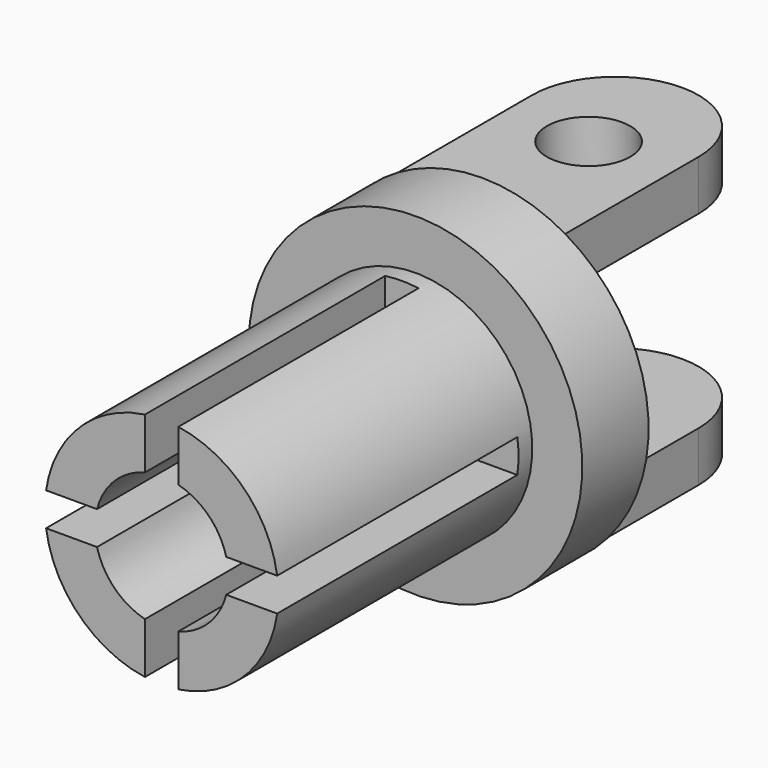
from build123d import *

# Parameters (mm, degrees)
F2_W     = 10
F2_H     = 3
F3_DEPTH = 15
F4_R     = 4.99999
F5_R     = 2.5
F6_DEPTH = 18.6612540378
F7_W     = 2
F7_H     = 4.8000003753
F7_W_2   = 4.8000003753
F7_H_2   = 2
F8_DEPTH = 18


# Not quite as in the source:
# - a fillet or chamfer is up to 0.001 mm smaller than in the source, because OpenCascade refuses the exact size


with BuildPart() as f1:
    # F0 (on Top) → F1 (revolve)
    with BuildSketch(Plane.XY):
        Polygon((0, 9.2748147342), (-10, 9.2748147342), (-10, 4.304778154), (-7, 4.304778154), (-7, -14.7251852658), (-4, -14.7251852658), (-4, 4.2748147342), (0, 4.2748147342), align=None)
    revolve(axis=Axis((0, 6.7748147342, 0), (0, -1, 0)))

    # F2 (on face) → F3 (join)
    with BuildSketch(Plane(origin=(0, 9.2748147342, 0), x_dir=(-1, 0, 0), z_dir=(0, 1, 0))):
        with Locations((0, 7.1602540378)):
            Rectangle(F2_W, F2_H)
        with Locations((0, -7.1602540378)):
            Rectangle(F2_W, F2_H)
    extrude(amount=F3_DEPTH)

    # F4 (radius 5 in the source; OpenCascade refuses exactly that, so slightly less here)
    f4_edges = [f1.edges().sort_by_distance(p)[0] for p in [
        (-5, 24.274815, -7.160254),
        (5, 24.274815, -7.160254),
        (5, 24.274815, 7.160254),
        (-5, 24.274815, 7.160254),
    ]]
    fillet(f4_edges, radius=F4_R)

    # F5 (on face) → F6 (cut, through all)
    with BuildSketch(Plane(origin=(0, 0, -8.6602540378), x_dir=(1, 0, 0), z_dir=(0, 0, -1))):
        with Locations((0, -17.2748147342)):
            Circle(F5_R)
    extrude(amount=-F6_DEPTH, mode=Mode.SUBTRACT)

    # F7 (on face) → F8 (cut)
    with BuildSketch(Plane.XZ.offset(14.7251852658)):
        with Locations((0, 5.4849120788)):
            Rectangle(F7_W, F7_H)
        with Locations((-5.4849120788, 0)):
            Rectangle(F7_W_2, F7_H_2)
        with Locations((0, -5.4849120788)):
            Rectangle(F7_W, F7_H)
        with Locations((5.4849120788, 0)):
            Rectangle(F7_W_2, F7_H_2)
    extrude(amount=-F8_DEPTH, mode=Mode.SUBTRACT)


solid = f1.part
